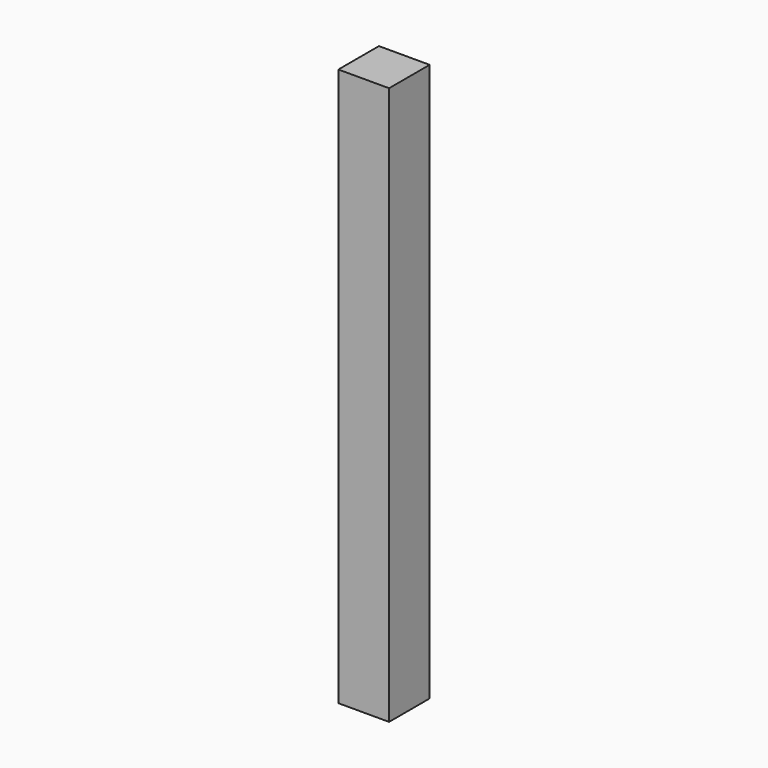
from build123d import *

# Parameters (mm, degrees)
F0_W          = 5
F0_H          = 55
F1_DEPTH      = 2.5
F1_DEPTH_BACK = 2.5


# Not quite as in the source:
# - the program builds the solid bodies; features that only make, move or delete a surface that nothing else refers to are left out


with BuildPart() as f1:
    # F0 (on Front) → F1 (new body, two sides)
    with BuildSketch(Plane.XZ) as f1_sk:
        Rectangle(F0_W, F0_H)
    extrude(amount=F1_DEPTH)
    extrude(f1_sk.sketch, amount=-F1_DEPTH_BACK)


solid = f1.part
